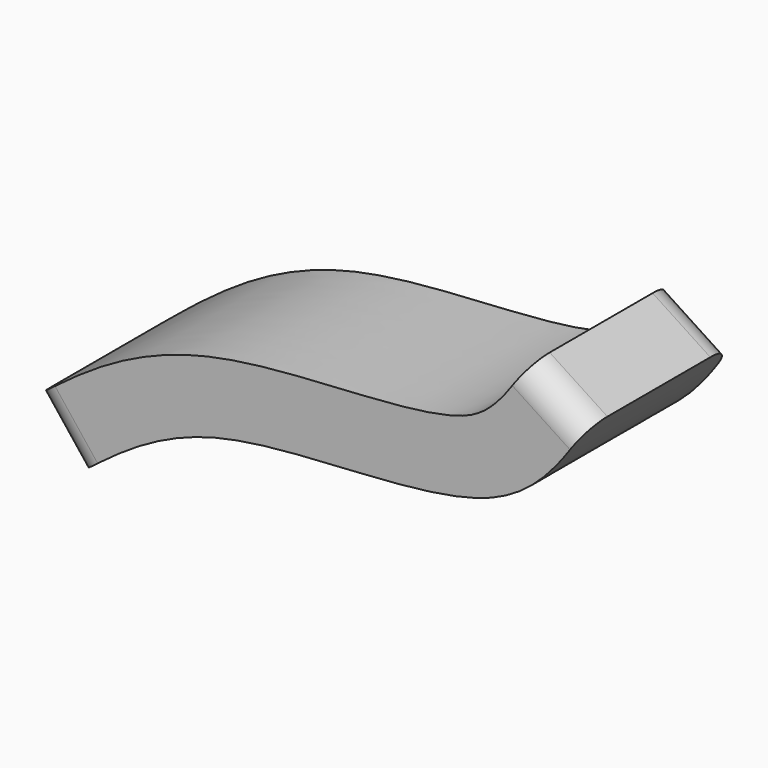
from build123d import *

# Parameters (mm, degrees)
F1_DEPTH = 50.8
F2_R     = 7.62


# Not quite as in the source:
# - the dataset's text gives a spline's control points without its knots; the knots are read off the source's solid


with BuildPart() as f1:
    # F0 (on Front) → F1 (new body)
    with BuildSketch(Plane.XZ):
        with BuildLine():
            Line((-99.140569867, 0.9624105209), (-87.3548537493, -14.0041988343))
            add(Edge.make_bspline(
                [(-87.3548537493, -14.0041988343), (-75.988278967, -5.0533923801), (-50.1295268695, 15.3095304535), (30.893884095, 8.2384364656), (46.8860391937, 32.7172550289), (53.4705743194, 42.7960492671)],
                knots=[0, 0, 0, 0, 0.3157202484, 0.7182578563, 1, 1, 1, 1], degree=3))
            Line((53.4705743194, 42.7960492671), (37.5223574351, 53.2151124789))
            add(Edge.make_bspline(
                [(-99.140569867, 0.9624105209), (-96.8904420168, 2.7343127228), (-92.1822042841, 6.4455239555), (-85.5235588099, 11.2675833523), (-79.5864663, 15.0368959025), (-74.7994531697, 17.76009584), (-69.6558135521, 20.3182414285), (-65.0611322891, 22.2609359989), (-61.1978217529, 23.6729575033), (-58.2065681515, 24.6544942334), (-55.1214837936, 25.5525626666), (-52.4729857991, 26.2270304858), (-50.3067006534, 26.719744138), (-48.1421714357, 27.1749366825), (-45.4314468519, 27.6813125017), (-42.1742127519, 28.2025864044), (-37.8269791769, 28.7994489886), (-32.3916532491, 29.3896702982), (-25.8983489378, 29.9250625326), (-19.4783594472, 30.3521259056), (-13.18669172, 30.728444081), (-7.0884593281, 31.106185302), (-1.2587690845, 31.5324500009), (4.2164339577, 32.0481157479), (9.2386519552, 32.6845781763), (12.9522070386, 33.3294214338), (15.5755953046, 33.9081226339), (17.3523919076, 34.3679262028), (18.6587604495, 34.7650514573), (19.5933067855, 35.0853518104), (20.2315125197, 35.3225581279), (20.8286299659, 35.5632785947), (21.5938847658, 35.8965263385), (22.4896769447, 36.3324178593), (23.4909840998, 36.8896341285), (24.7523369479, 37.6841668244), (26.2358104686, 38.7907897037), (27.9729819139, 40.3658338924), (29.7289492605, 42.2472254179), (31.5360340689, 44.4701786628), (34.0424131946, 47.8999932909), (36.0616833593, 50.9792927623), (37.5223574351, 53.2151124789)],
                knots=[0, 0, 0, 0, 0.0625, 0.125, 0.15625, 0.1875, 0.21875, 0.25, 0.265625, 0.28125, 0.296875, 0.3125, 0.3203125, 0.328125, 0.34375, 0.359375, 0.375, 0.40625, 0.4375, 0.46875, 0.5, 0.53125, 0.5625, 0.59375, 0.625, 0.65625, 0.671875, 0.6875, 0.703125, 0.7109375, 0.71875, 0.7265625, 0.734375, 0.75, 0.765625, 0.78125, 0.8125, 0.84375, 0.875, 0.90625, 0.9375, 1, 1, 1, 1], degree=3))
        make_face()
    extrude(amount=F1_DEPTH)

    # F2
    f2_edges = [f1.edges().sort_by_distance(p)[0] for p in [
        (45.496466, -50.8, 48.005581),
        (-93.247712, -50.8, -6.520894),
        (-93.247712, 0, -6.520894),
        (45.496466, 0, 48.005581),
    ]]
    fillet(f2_edges, radius=F2_R)


solid = f1.part
